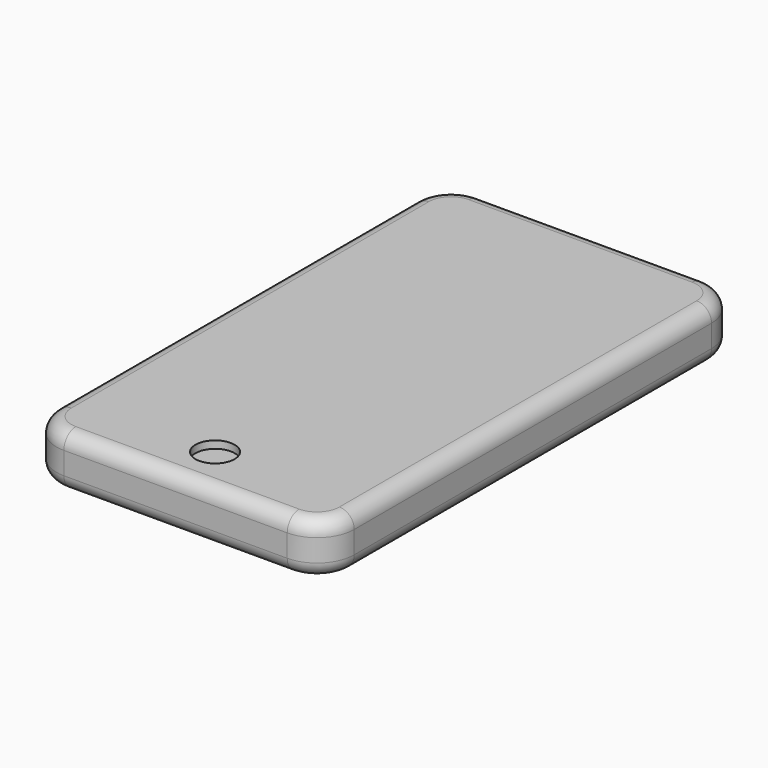
from build123d import *

# Parameters (mm, degrees)
F0_W         = 40
F0_H         = 70
F1_DEPTH     = 7
F2_R         = 5
F3_R         = 2
F4_DEPTH     = 3
F5_T1_DEPTH  = 60
F5_T3_DEPTH  = 30
F5_T6_ANGLE  = 90
F5_T8_ANGLE  = 90
F5_T10_ANGLE = 90
F5_T12_ANGLE = 90
F5_T14_ANGLE = 90
F5_T16_ANGLE = 90
F5_T18_ANGLE = 90
F5_T20_ANGLE = 90
F6_R         = 2.6271107644
F7_DEPTH     = 1


# Not quite as in the source:
# - a fillet or chamfer that OpenCascade refuses, or shapes differently, is made with other operations: its cross-section is extruded or revolved along the edge and cut away or added


with BuildPart() as f1:
    # F0 (on Top) → F1 (new body)
    with BuildSketch(Plane.XY):
        with Locations((20, 35)):
            Rectangle(F0_W, F0_H)
    extrude(amount=F1_DEPTH)

    # F2
    f2_edges = [f1.edges().sort_by_distance(p)[0] for p in [
        (40, 70, 3.5),
        (0, 70, 3.5),
        (40, 0, 3.5),
        (0, 0, 3.5),
    ]]
    fillet(f2_edges, radius=F2_R)

    # F3 (on face) → F4 (cut)
    with BuildSketch(Plane(origin=(0, 70, 0), x_dir=(-1, 0, 0), z_dir=(0, 1, 0))):
        with Locations((-29.8281734893, 3.5)):
            Circle(F3_R)
    extrude(amount=-F4_DEPTH, mode=Mode.SUBTRACT)

    # F5: fillet of radius 2 on 16 edges, made by hand

    # F5_s2 → F5_t1 (cut)
    with BuildSketch(Plane.XZ.offset(-65)):
        with BuildLine():
            ThreePointArc((0, 5), (0.5857864376, 6.4142135624), (2, 7))
            Line((2, 7), (0, 7))
            Line((0, 7), (0, 5))
        make_face()
        with BuildLine():
            ThreePointArc((0, 2), (0.5857864376, 0.5857864376), (2, 0))
            Line((2, 0), (0, 0))
            Line((0, 0), (0, 2))
        make_face()
        with BuildLine():
            ThreePointArc((38, 0), (39.4142135624, 0.5857864376), (40, 2))
            Line((40, 2), (40, 0))
            Line((40, 0), (38, 0))
        make_face()
        with BuildLine():
            ThreePointArc((38, 7), (39.4142135624, 6.4142135624), (40, 5))
            Line((40, 5), (40, 7))
            Line((40, 7), (38, 7))
        make_face()
    extrude(amount=F5_T1_DEPTH, mode=Mode.SUBTRACT)

    # F5_s4 → F5_t3 (cut)
    with BuildSketch(Plane.YZ.offset(5)):
        with BuildLine():
            ThreePointArc((68, 0), (69.4142135624, 0.5857864376), (70, 2))
            Line((70, 2), (70, 0))
            Line((70, 0), (68, 0))
        make_face()
        with BuildLine():
            ThreePointArc((2, 0), (0.5857864376, 0.5857864376), (0, 2))
            Line((0, 2), (0, 0))
            Line((0, 0), (2, 0))
        make_face()
        with BuildLine():
            ThreePointArc((68, 7), (69.4142135624, 6.4142135624), (70, 5))
            Line((70, 5), (70, 7))
            Line((70, 7), (68, 7))
        make_face()
        with BuildLine():
            ThreePointArc((2, 7), (0.5857864376, 6.4142135624), (0, 5))
            Line((0, 5), (0, 7))
            Line((0, 7), (2, 7))
        make_face()
    extrude(amount=F5_T3_DEPTH, mode=Mode.SUBTRACT)

    # F5_s5 → F5_t6 (revolve, cut)
    with BuildSketch(Plane.XZ.offset(-65)):
        with BuildLine():
            ThreePointArc((2, 0), (0.5857864376, 0.5857864376), (0, 2))
            Line((0, 2), (0, 0))
            Line((0, 0), (2, 0))
        make_face()
    revolve(axis=Axis((5, 65, 0), (0, 0, -1)), revolution_arc=F5_T6_ANGLE, mode=Mode.SUBTRACT)

    # F5_s7 → F5_t8 (revolve, cut)
    with BuildSketch(Plane.XZ.offset(-5)):
        with BuildLine():
            ThreePointArc((2, 0), (0.5857864376, 0.5857864376), (0, 2))
            Line((0, 2), (0, 0))
            Line((0, 0), (2, 0))
        make_face()
    revolve(axis=Axis((5, 5, 0), (0, 0, 1)), revolution_arc=F5_T8_ANGLE, mode=Mode.SUBTRACT)

    # F5_s9 → F5_t10 (revolve, cut)
    with BuildSketch(Plane.XZ.offset(-65)):
        with BuildLine():
            ThreePointArc((38, 0), (39.4142135624, 0.5857864376), (40, 2))
            Line((40, 2), (40, 0))
            Line((40, 0), (38, 0))
        make_face()
    revolve(axis=Axis((35, 65, 0), (0, 0, 1)), revolution_arc=F5_T10_ANGLE, mode=Mode.SUBTRACT)

    # F5_s11 → F5_t12 (revolve, cut)
    with BuildSketch(Plane.YZ.offset(35)):
        with BuildLine():
            ThreePointArc((2, 0), (0.5857864376, 0.5857864376), (0, 2))
            Line((0, 2), (0, 0))
            Line((0, 0), (2, 0))
        make_face()
    revolve(axis=Axis((35, 5, 0), (0, 0, 1)), revolution_arc=F5_T12_ANGLE, mode=Mode.SUBTRACT)

    # F5_s13 → F5_t14 (revolve, cut)
    with BuildSketch(Plane.XZ.offset(-65)):
        with BuildLine():
            ThreePointArc((0, 5), (0.5857864376, 6.4142135624), (2, 7))
            Line((2, 7), (0, 7))
            Line((0, 7), (0, 5))
        make_face()
    revolve(axis=Axis((5, 65, 7), (0, 0, -1)), revolution_arc=F5_T14_ANGLE, mode=Mode.SUBTRACT)

    # F5_s15 → F5_t16 (revolve, cut)
    with BuildSketch(Plane.XZ.offset(-5)):
        with BuildLine():
            ThreePointArc((0, 5), (0.5857864376, 6.4142135624), (2, 7))
            Line((2, 7), (0, 7))
            Line((0, 7), (0, 5))
        make_face()
    revolve(axis=Axis((5, 5, 7), (0, 0, 1)), revolution_arc=F5_T16_ANGLE, mode=Mode.SUBTRACT)

    # F5_s17 → F5_t18 (revolve, cut)
    with BuildSketch(Plane.XZ.offset(-65)):
        with BuildLine():
            ThreePointArc((38, 7), (39.4142135624, 6.4142135624), (40, 5))
            Line((40, 5), (40, 7))
            Line((40, 7), (38, 7))
        make_face()
    revolve(axis=Axis((35, 65, 7), (0, 0, 1)), revolution_arc=F5_T18_ANGLE, mode=Mode.SUBTRACT)

    # F5_s19 → F5_t20 (revolve, cut)
    with BuildSketch(Plane.YZ.offset(35)):
        with BuildLine():
            ThreePointArc((2, 7), (0.5857864376, 6.4142135624), (0, 5))
            Line((0, 5), (0, 7))
            Line((0, 7), (2, 7))
        make_face()
    revolve(axis=Axis((35, 5, 7), (0, 0, 1)), revolution_arc=F5_T20_ANGLE, mode=Mode.SUBTRACT)

    # F6 (on face) → F7 (cut)
    with BuildSketch(Plane.XY.offset(7)):
        with Locations((20, 6.6271107644)):
            Circle(F6_R)
    extrude(amount=-F7_DEPTH, mode=Mode.SUBTRACT)


solid = f1.part
